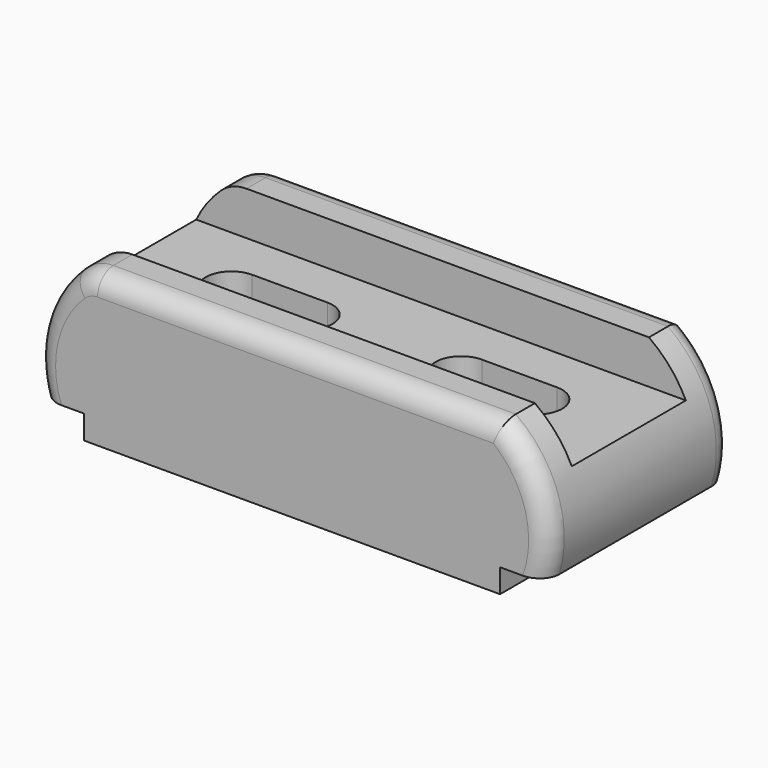
from build123d import *

# Parameters (mm, degrees)
F1_DEPTH = 58
F2_W     = 21.7170343468
F2_H     = 36
F2_W_2   = 18.1216797089
F2_W_3   = 101.6265741507
F3_DEPTH = 11
F5_DEPTH = 27
F6_DEPTH = 27
F7_R     = 5
F8_R     = 5


# Not quite as in the source:
# - a feature names something its author has since deleted; it is built from what else it names


with BuildPart() as f1:
    # F0 (on Front) → F1 (new body)
    with BuildSketch(Plane.XZ):
        with BuildLine():
            Line((0, 6), (0, 0))
            Line((0, 0), (105, 0))
            Line((105, 0), (105, 6))
            Line((105, 6), (116, 6))
            ThreePointArc((116, 6), (115.651030618, 23.7706667749), (105, 38))
            Line((105, 38), (3.3734258493, 38))
            ThreePointArc((3.3734258493, 38), (-0.1544899089, 37.3225666374), (-3.1805835495, 35.3866268563))
            ThreePointArc((-3.1805835495, 35.3866268563), (-11.2509687534, 21.8004179002), (-11, 6))
            Line((-11, 6), (0, 6))
        make_face()
    extrude(amount=-F1_DEPTH)

    # F2 (on face) → F3 (cut)
    with BuildSketch(Plane.XY.offset(38)):
        with Locations((115.8585171734, 29)):
            Rectangle(F2_W, F2_H)
        with Locations((-5.6874140052, 29)):
            Rectangle(F2_W_2, F2_H)
        with Locations((54.1867129246, 29)):
            Rectangle(F2_W_3, F2_H)
    extrude(amount=-F3_DEPTH, mode=Mode.SUBTRACT)

    # F4 (on face) → F5 (cut)
    with BuildSketch(Plane.XY.offset(27)):
        with BuildLine():
            Line((33, 35.5), (14, 35.5))
            ThreePointArc((14, 35.5), (7.5, 29), (14, 22.5))
            Line((14, 22.5), (33, 22.5))
            ThreePointArc((33, 22.5), (39.5, 29), (33, 35.5))
        make_face()
    extrude(amount=-F5_DEPTH, mode=Mode.SUBTRACT)

    # F4 (on face) → F6 (cut)
    with BuildSketch(Plane.XY.offset(27)):
        with BuildLine():
            Line((91, 35.5), (72, 35.5))
            ThreePointArc((72, 35.5), (65.5, 29), (72, 22.5))
            Line((72, 22.5), (91, 22.5))
            ThreePointArc((91, 22.5), (97.5, 29), (91, 35.5))
        make_face()
    extrude(amount=-F6_DEPTH, mode=Mode.SUBTRACT)

    # F7
    f7_edges = [f1.edges().sort_by_distance(p)[0] for p in [
        (54.186713, 0, 38),
        (115.651031, 0, 23.770667),
    ]]
    fillet(f7_edges, radius=F7_R)

    # F8
    f8_edges = [f1.edges().sort_by_distance(p)[0] for p in [
        (115.651031, 58, 23.770667),
        (54.186713, 58, 38),
    ]]
    fillet(f8_edges, radius=F8_R)


solid = f1.part
